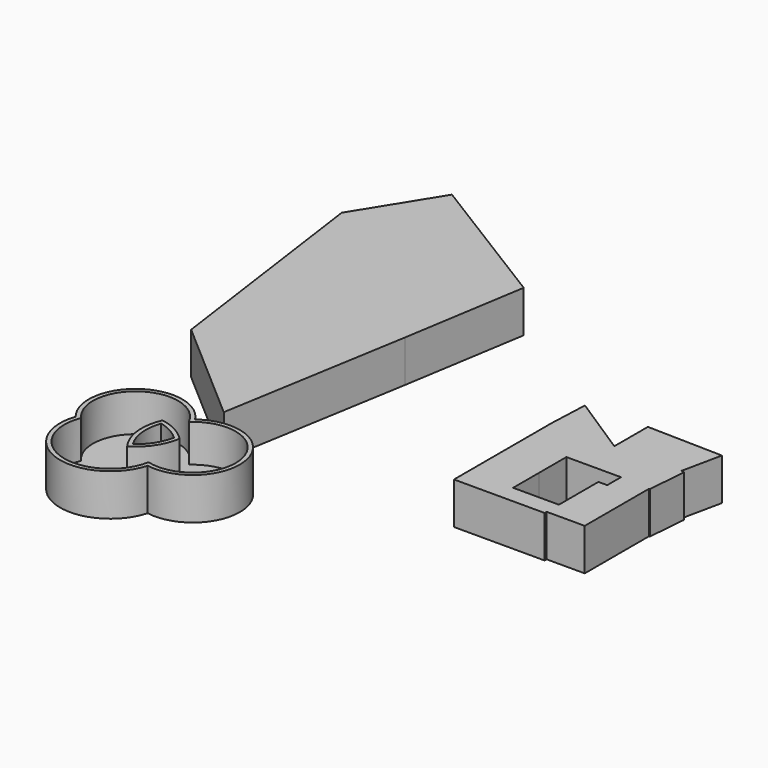
from build123d import *

# Parameters (mm, degrees)
F1_DEPTH = 25.4
F3_DEPTH = 25.4
F4_T     = -2.54
F5_W     = 27.2268103436
F5_H     = 10.8409523964
F5_W_2   = 23.1075808406
F5_H_2   = 9.3090385199
F5_H_3   = 6.7053586245
F5_H_4   = 12.9625052214
F6_DEPTH = 25.4
F7_T     = -2.54


# Not quite as in the source:
# - ends of sketch curves that miss each other by under 0.0002 mm in the source are joined


with BuildPart() as f1:
    # F0 (on Top) → F1 (new body)
    with BuildSketch(Plane.XY):
        Polygon((-156.3564315383, 1.9787269735), (-188.787728548, -95.9389954805), (-123.7907707691, -152.4280905724), (-104.6589389443, -39.0103124082), (-155.8479517698, 0), align=None)
        Polygon((-208.030372858, 42.3308461905), (-188.787728548, -95.9389954805), (-156.3564315383, 1.9787269735), (-178.8411438465, 89.4770100713), align=None)
        Polygon((-178.8411438465, 89.4770100713), (-156.3564315383, 1.9787269735), (-155.8479517698, 0), (-104.6589389443, -39.0103124082), (-92.5675530585, 36.0631288163), align=None)
    extrude(amount=F1_DEPTH)

    # F4
    f4_openings = [f1.faces().sort_by_distance(p)[0] for p in [
        (-151.431533, -21.743428, 0),
    ]]
    offset(amount=F4_T, openings=f4_openings)


with BuildPart() as f3:
    # F2 (on Top) → F3 (new body)
    with BuildSketch(Plane.XY):
        with BuildLine():
            ThreePointArc((-125.8460203447, -187.6461548391), (-125.4230402026, -184.8440134333), (-125.2815768128, -182.0136606693))
            ThreePointArc((-125.2815768128, -182.0136606693), (-126.4221290125, -174.0482010322), (-129.7521277548, -166.7228672564))
            ThreePointArc((-129.7521277548, -166.7228672564), (-135.6943033651, -172.6451210363), (-139.658973853, -180.0386268854))
            ThreePointArc((-139.658973853, -180.0386268854), (-132.2511693873, -182.9321324426), (-125.8460203447, -187.6461548391))
        make_face()
        with BuildLine():
            ThreePointArc((-129.7521277548, -166.7228672564), (-126.4221290125, -174.0482010322), (-125.2815768128, -182.0136606693))
            ThreePointArc((-125.2815768128, -182.0136606693), (-125.4230402026, -184.8440134333), (-125.8460203447, -187.6461548391))
            ThreePointArc((-125.8460203447, -187.6461548391), (-118.9342268143, -197.6635782995), (-116.5005442713, -209.5882943076))
            ThreePointArc((-116.5005442713, -209.5882943076), (-116.7862081683, -213.7481993276), (-117.637836757, -217.8300055925))
            ThreePointArc((-117.637836757, -217.8300055925), (-94.3883375859, -211.5305918967), (-84.2287479373, -189.6901577711))
            ThreePointArc((-84.2287479373, -189.6901577711), (-99.9217410648, -164.1956753112), (-129.7521277548, -166.7228672564))
        make_face()
        with BuildLine():
            ThreePointArc((-139.658973853, -180.0386268854), (-135.6943033651, -172.6451210363), (-129.7521277548, -166.7228672564))
            ThreePointArc((-129.7521277548, -166.7228672564), (-170.2484998371, -158.9754699319), (-175.7588912266, -199.8363791712))
            ThreePointArc((-175.7588912266, -199.8363791712), (-161.5652178843, -182.9058167896), (-139.658973853, -180.0386268854))
        make_face()
        with BuildLine():
            ThreePointArc((-116.5005442713, -209.5882943076), (-118.9342268143, -197.6635782995), (-125.8460203447, -187.6461548391))
            ThreePointArc((-125.8460203447, -187.6461548391), (-129.7681307705, -197.3294537383), (-136.9277512541, -204.9379399409))
            ThreePointArc((-136.9277512541, -204.9379399409), (-128.6511581783, -213.4314047769), (-117.637836757, -217.8300055925))
            ThreePointArc((-117.637836757, -217.8300055925), (-116.7862081683, -213.7481993276), (-116.5005442713, -209.5882943076))
        make_face()
        with BuildLine():
            ThreePointArc((-139.658973853, -180.0386268854), (-161.5652178843, -182.9058167896), (-175.7588912266, -199.8363791712))
            ThreePointArc((-175.7588912266, -199.8363791712), (-157.3640992757, -210.1569336627), (-136.9277512541, -204.9379399409))
            ThreePointArc((-136.9277512541, -204.9379399409), (-141.1692469428, -192.8037411296), (-139.658973853, -180.0386268854))
        make_face()
        with BuildLine():
            ThreePointArc((-136.9277512541, -204.9379399409), (-157.3640992757, -210.1569336627), (-175.7588912266, -199.8363791712))
            ThreePointArc((-175.7588912266, -199.8363791712), (-155.9319849015, -238.6586300828), (-117.637836757, -217.8300055925))
            ThreePointArc((-117.637836757, -217.8300055925), (-128.6511581783, -213.4314047769), (-136.9277512541, -204.9379399409))
        make_face()
    extrude(amount=F3_DEPTH)

    # F7
    f7_openings = [f3.faces().sort_by_distance(p)[0] for p in [
        (-169.486097, -160.034726, 25.4),
    ]]
    offset(amount=F7_T, openings=f7_openings, kind=Kind.INTERSECTION)


with BuildPart() as f6:
    # F5 (on Top) → F6 (new body)
    with BuildSketch(Plane.XY):
        Polygon((4.5195547864, -64.0997934229), (42.5464881825, -64.0997934229), (23.116490582, -51.49882088), align=None)
        Polygon((4.5195547864, -97.3955392838), (31.7463651299, -97.3955392838), (31.7463651299, -86.9494602084), align=None)
        Polygon((5.5383988656, -40.0988683105), (4.5195547864, -64.0997934229), (23.116490582, -51.49882088), align=None)
        Polygon((59.5347508788, -62.1402259879), (42.5464881825, -64.0997934229), (83.1468105316, -64.0997934229), (83.1517481659, -64.0764903684), align=None)
        with Locations((18.1329599582, -132.7852457762)):
            Rectangle(F5_W, F5_H)
        Polygon((64.8705512285, -97.3955392838), (82.6423317194, -97.3955392838), (64.8705512285, -86.9494602084), align=None)
        Polygon((59.5347508788, -107.6969057322), (82.6423317194, -107.6969057322), (82.6423317194, -97.3955392838), (64.8705512285, -97.3955392838), (59.5347508788, -97.3955392838), align=None)
        Polygon((59.5347508788, -136.6738080978), (59.5347508788, -127.364769578), (31.7463651299, -127.364769578), (31.7463651299, -138.2057219744), (59.5347508788, -138.2057219744), align=None)
        with Locations((71.0885412991, -132.0192888379)):
            Rectangle(F5_W_2, F5_H_2)
        with Locations((18.1329599582, -124.0120902658)):
            Rectangle(F5_W, F5_H_3)
        Polygon((64.8705512285, -86.9494602084), (82.6423317194, -97.3955392838), (82.6423317194, -87.9362548824), align=None)
        with Locations((71.0885412991, -114.1781583428)):
            Rectangle(F5_W_2, F5_H_4)
        with Locations((71.0885412991, -124.0120902658)):
            Rectangle(F5_W_2, F5_H_3)
        Polygon((82.6423317194, -87.6677388178), (82.6423317194, -87.9362548824), (83.1468105316, -87.9642665386), align=None)
        Polygon((4.5195547864, -107.6969057322), (31.7463651299, -107.6969057322), (31.7463651299, -97.3955392838), (4.5195547864, -97.3955392838), (4.5195547864, -102.546222508), align=None)
        with Locations((18.1329599582, -114.1781583428)):
            Rectangle(F5_W, F5_H_4)
        Polygon((42.5464881825, -64.0997934229), (82.6423317194, -87.6677388178), (83.1468105316, -87.9642665386), (85.0922316313, -64.2355829477), (83.1517481659, -64.0764903684), (83.1468105316, -64.0997934229), align=None)
        Polygon((4.5195547864, -86.9494602084), (6.1366017055, -86.9494602084), (42.5464881825, -64.0997934229), (4.5195547864, -64.0997934229), align=None)
        Polygon((31.7463651299, -86.9494602084), (64.8705512285, -86.9494602084), (82.6423317194, -87.9362548824), (82.6423317194, -87.6677388178), (42.5464881825, -64.0997934229), (6.1366017055, -86.9494602084), align=None)
        Polygon((4.5195547864, -87.9642665386), (6.1366017055, -86.9494602084), (4.5195547864, -86.9494602084), align=None)
        Polygon((4.5195547864, -97.3955392838), (31.7463651299, -86.9494602084), (6.1366017055, -86.9494602084), (4.5195547864, -87.9642665386), align=None)
        Polygon((42.5464881825, -38.6408381164), (42.5464881825, -64.0997934229), (59.5347508788, -62.1402259879), (83.1517481659, -64.0764903684), (88.3195400238, -39.6872125566), align=None)
    extrude(amount=F6_DEPTH)


solid = Compound([f1.part, f3.part, f6.part])
